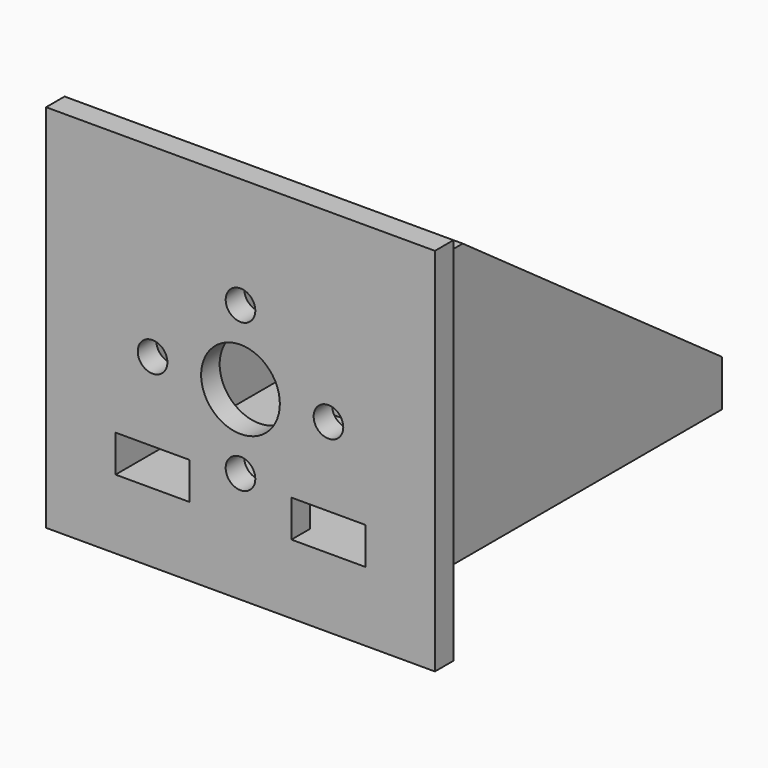
from build123d import *

# Parameters (mm, degrees)
F0_W      = 32
F0_H      = 30
F1_DEPTH  = 45
F2_T      = -2.5
F4_DEPTH  = 32.001
F5_W      = 42
F5_H      = 40
F6_DEPTH  = 2.5
F7_R      = 1.6
F7_R_2    = 4.25
F7_W      = 8
F7_H      = 4
F8_DEPTH  = 45.001
F9_W      = 15
F9_H      = 25
F10_DEPTH = 3
F11_R     = 5
F12_DEPTH = 2


# Not quite as in the source:
# - a fillet or chamfer that OpenCascade refuses, or shapes differently, is made with other operations: its cross-section is extruded or revolved along the edge and cut away or added


with BuildPart() as f1:
    # F0 (on Front) → F1 (new body)
    with BuildSketch(Plane.XZ):
        Rectangle(F0_W, F0_H)
    extrude(amount=-F1_DEPTH)

    # F2
    f2_openings = [f1.faces().sort_by_distance(p)[0] for p in [
        (0, 45, 0),
    ]]
    offset(amount=F2_T, openings=f2_openings)

    # F3 (on face) → F4 (cut, through all)
    with BuildSketch(Plane.YZ.offset(16)):
        Polygon((45, 15), (10, 15), (45, -10), align=None)
    extrude(amount=-F4_DEPTH, mode=Mode.SUBTRACT)

    # F5 (on face) → F6 (join)
    with BuildSketch(Plane.XZ):
        Rectangle(F5_W, F5_H)
    extrude(amount=-F6_DEPTH)

    # F7 (on face) → F8 (cut, through all)
    with BuildSketch(Plane.XZ):
        with Locations((9.5, 0)):
            Circle(F7_R)
        with Locations((-9.5, 0)):
            Circle(F7_R)
        with Locations((0, -8)):
            Circle(F7_R)
        with Locations((0, 8)):
            Circle(F7_R)
        Circle(F7_R_2)
        with Locations((9.5, -10.5)):
            Rectangle(F7_W, F7_H)
        with Locations((-9.5, -10.5)):
            Rectangle(F7_W, F7_H)
    extrude(amount=-F8_DEPTH, mode=Mode.SUBTRACT)

    # F9 (on face) → F10 (join)
    with BuildSketch(Plane.XY.offset(-12.5)):
        with Locations((0, 32.5)):
            Rectangle(F9_W, F9_H)
    extrude(amount=F10_DEPTH)

    # F11 (on face) → F12 (cut)
    with BuildSketch(Plane(origin=(0, 0, -15), x_dir=(1, 0, 0), z_dir=(0, 0, -1))):
        with Locations((0, -28)):
            Circle(F11_R)
    extrude(amount=-F12_DEPTH, mode=Mode.SUBTRACT)

    # F13: fillet of radius 5 on 1 edges, made by hand

    # F13_s1 → F13_t2 (revolve)
    with BuildSketch(Plane.XZ.offset(-28)):
        with BuildLine():
            ThreePointArc((5, -15), (3.2360679775, -13.527864045), (1, -13))
            Line((1, -13), (5, -13))
            Line((5, -13), (5, -15))
        make_face()
    revolve(axis=Axis((0, 28, -13), (0, 0, -1)))


solid = f1.part
